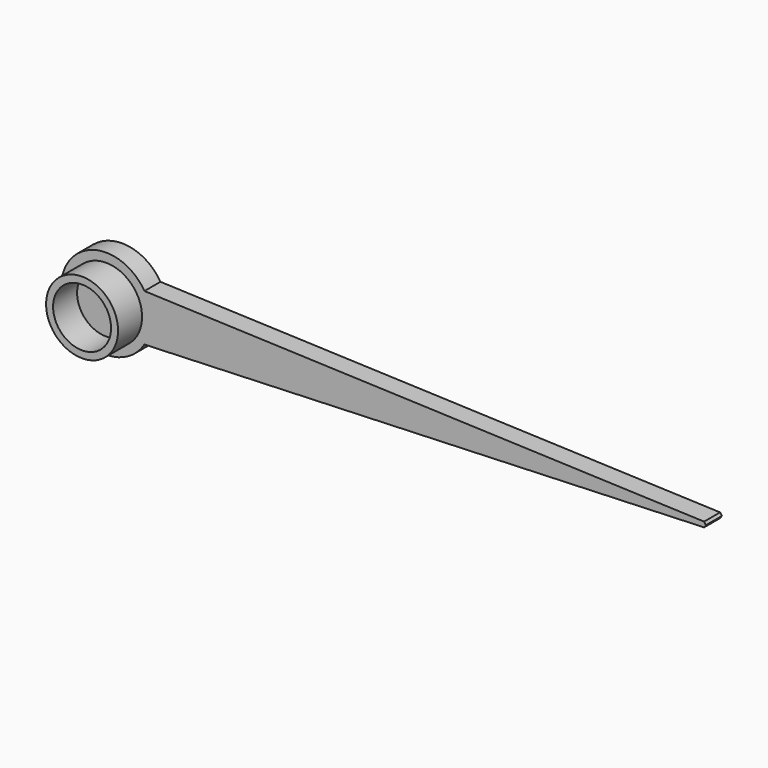
from build123d import *

# Parameters (mm, degrees)
F1_DEPTH = 1
F2_R     = 3.6
F2_R_2   = 2.9
F3_DEPTH = 5
F4_DEPTH = 1


with BuildPart() as f1:
    # F0 (on Front) → F1 (new body, symmetric)
    with BuildSketch(Plane.XZ):
        with BuildLine():
            ThreePointArc((3.8359832735, -2.3527074457), (4.3308154389, -1.2223083222), (4.5, 0))
            ThreePointArc((4.5, 0), (4.3308154389, 1.2223083222), (3.8359832735, 2.3527074457))
            ThreePointArc((3.8359832735, 2.3527074457), (-4.5, 0), (3.8359832735, -2.3527074457))
        make_face()
        with BuildLine():
            ThreePointArc((3.8359832735, 2.3527074457), (4.3308154389, 1.2223083222), (4.5, 0))
            ThreePointArc((4.5, 0), (4.3308154389, -1.2223083222), (3.8359832735, -2.3527074457))
            Line((3.8359832735, -2.3527074457), (59.7996972501, -0.2551520593))
            Line((59.7996972501, -0.2551520593), (59.9825401634, -9.9e-09))
            Line((59.9825401634, -9.9e-09), (59.7996972501, 0.2551520395))
            Line((59.7996972501, 0.2551520395), (3.8359832735, 2.3527074457))
        make_face()
    extrude(amount=F1_DEPTH, both=True)

    # F2 (on face) → F3 (join)
    with BuildSketch(Plane(origin=(0, 1, 0), x_dir=(-1, 0, 0), z_dir=(0, 1, 0))):
        Circle(F2_R)
        Circle(F2_R_2, mode=Mode.SUBTRACT)
    extrude(amount=-F3_DEPTH)

    # F0 (on Front) → F4 (join, symmetric)
    with BuildSketch(Plane.XZ):
        with BuildLine():
            ThreePointArc((3.8359832735, 2.3527074457), (4.3308154389, 1.2223083222), (4.5, 0))
            ThreePointArc((4.5, 0), (4.3308154389, -1.2223083222), (3.8359832735, -2.3527074457))
            Line((3.8359832735, -2.3527074457), (59.7996972501, -0.2551520593))
            Line((59.7996972501, -0.2551520593), (59.9825401634, -9.9e-09))
            Line((59.9825401634, -9.9e-09), (59.7996972501, 0.2551520395))
            Line((59.7996972501, 0.2551520395), (3.8359832735, 2.3527074457))
        make_face()
    extrude(amount=F4_DEPTH, both=True)


solid = f1.part
